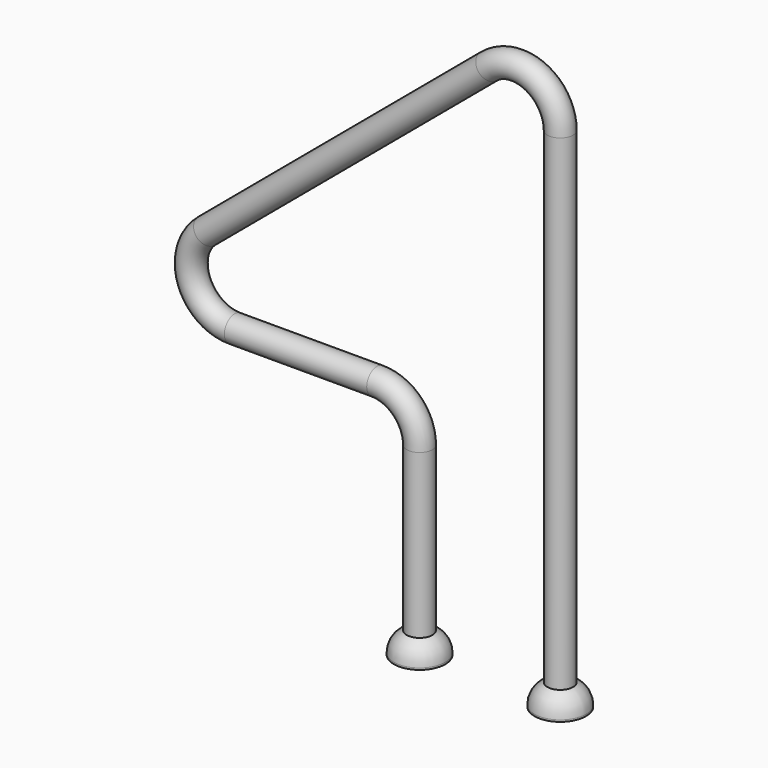
from build123d import *

# Parameters (mm, degrees)
F2_R     = 2.9933814251
F4_R     = 5.9933814251
F5_DEPTH = 5


# Not quite as in the source:
# - a fillet or chamfer that OpenCascade refuses, or shapes differently, is made with other operations: its cross-section is extruded or revolved along the edge and cut away or added


with BuildPart() as f3:
    # F3: sweep along a path in F0
    with BuildLine(Plane.XZ) as f3_path:
        Line((51.9430634924, -22.1786051989), (51.9430634924, 95.8719234608))
        ThreePointArc((51.9430634924, 95.8719234608), (46.1700643013, 104.9346197572), (35.5165706601, 103.533528376))
        Line((35.5165706601, 103.533528376), (-30.1489816492, 48.4537890892))
        ThreePointArc((-30.1489816492, 48.4537890892), (-33.11972376, 37.3728311031), (-23.7224888169, 30.7921841741))
        Line((-23.7224888169, 30.7921841741), (9.4017067552, 30.7921841741))
        ThreePointArc((9.4017067552, 30.7921841741), (16.472774567, 27.8632519859), (19.4017067552, 20.7921841741))
        Line((19.4017067552, 20.7921841741), (19.4017067552, -22.1786051989))
    # F2 (on line) → F3 (sweep)
    with BuildSketch(Plane.XY.offset(-22.1786051989)):
        with Locations((52.0414784551, 0)):
            Circle(F2_R)
    sweep(path=f3_path.line)

    # F4 (on line) → F5 (join)
    with BuildSketch(Plane.XY.offset(-22.1786051989)):
        with Locations((52.0414784551, 0)):
            Circle(F4_R)
        with Locations((19.3032917925, 0)):
            Circle(F4_R)
    extrude(amount=F5_DEPTH)

    # F6: fillet of radius 5 on 2 edges, made by hand

    # F6_s1 → F6_t2 (revolve, cut)
    with BuildSketch(Plane.XZ):
        with BuildLine():
            ThreePointArc((58.0348598802, -21.7611808938), (57.2181600129, -19.0225681063), (55.0348598802, -17.1786051989))
            Line((55.0348598802, -17.1786051989), (58.0348598802, -17.1786051989))
            Line((58.0348598802, -17.1786051989), (58.0348598802, -21.7611808938))
        make_face()
    revolve(axis=Axis((52.0414784551, 0, -17.1786051989), (0, 0, 1)), mode=Mode.SUBTRACT)

    # F6_s3 → F6_t4 (revolve, cut)
    with BuildSketch(Plane.XZ):
        with BuildLine():
            ThreePointArc((22.2966732176, -17.1786051989), (24.4799733503, -19.0225681063), (25.2966732176, -21.7611808938))
            Line((25.2966732176, -21.7611808938), (25.2966732176, -17.1786051989))
            Line((25.2966732176, -17.1786051989), (22.2966732176, -17.1786051989))
        make_face()
    revolve(axis=Axis((19.3032917925, 0, -17.1786051989), (0, 0, 1)), mode=Mode.SUBTRACT)


solid = f3.part
